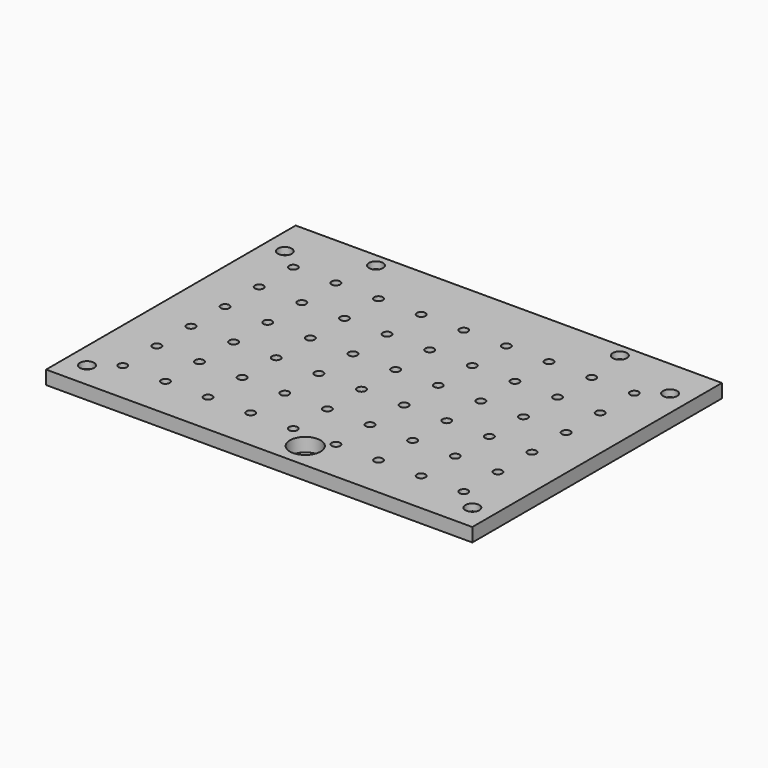
from build123d import *

# Parameters (mm, degrees)
F0_W           = 250
F0_H           = 183
F1_DEPTH       = 8
F3_D           = 4.4
F3_CBORE_D     = 8.25
F3_CBORE_DEPTH = 4
F4_D           = 18
F5_D           = 5


# Not quite as in the source:
# - a feature names something its author has since deleted; it is built from what else it names


with BuildPart() as f1:
    # F0 (on Top) → F1 (new body)
    with BuildSketch(Plane.XY):
        Rectangle(F0_W, F0_H)
    extrude(amount=F1_DEPTH)

    # F3 (through all)
    with Locations(Plane.XY.offset(8)):
        with Locations((-113, 68.5), (-113, -76.5), (113, -76.5), (113, 68.5), (71.5, 83.5), (-71.5, 83.5)):
            CounterBoreHole(F3_D / 2, F3_CBORE_D / 2, F3_CBORE_DEPTH)

    # F4 (through all)
    with Locations(Plane.XY.offset(8)):
        with Locations((15, -76.5)):
            Hole(F4_D / 2)

    # F5 (through all)
    with Locations(Plane.XY.offset(8)):
        with Locations((100, 58.5), (100, 33.5), (100, 8.5), (100, -16.5), (100, -41.5), (100, -66.5), (75, -66.5), (75, -41.5), (75, -16.5), (75, 8.5), (75, 33.5), (75, 58.5), (50, 58.5), (50, 33.5), (50, 8.5), (50, -16.5), (50, -41.5), (50, -66.5), (25, -66.5), (0, -66.5), (-25, -66.5), (-50, -66.5), (-75, -66.5), (-100, -66.5), (-100, -41.5), (-75, -41.5), (-50, -41.5), (-25, -41.5), (0, -41.5), (25, -41.5), (25, -16.5), (0, -16.5), (-25, -16.5), (-50, -16.5), (-75, -16.5), (-100, -16.5), (-100, 8.5), (-75, 8.5), (-50, 8.5), (-25, 8.5), (0, 8.5), (25, 8.5), (25, 33.5), (0, 33.5), (-25, 33.5), (-50, 33.5), (-75, 33.5), (-100, 33.5), (-100, 58.5), (-75, 58.5), (-50, 58.5), (25, 58.5), (-25, 58.5), (0, 58.5)):
            Hole(F5_D / 2)


solid = f1.part
